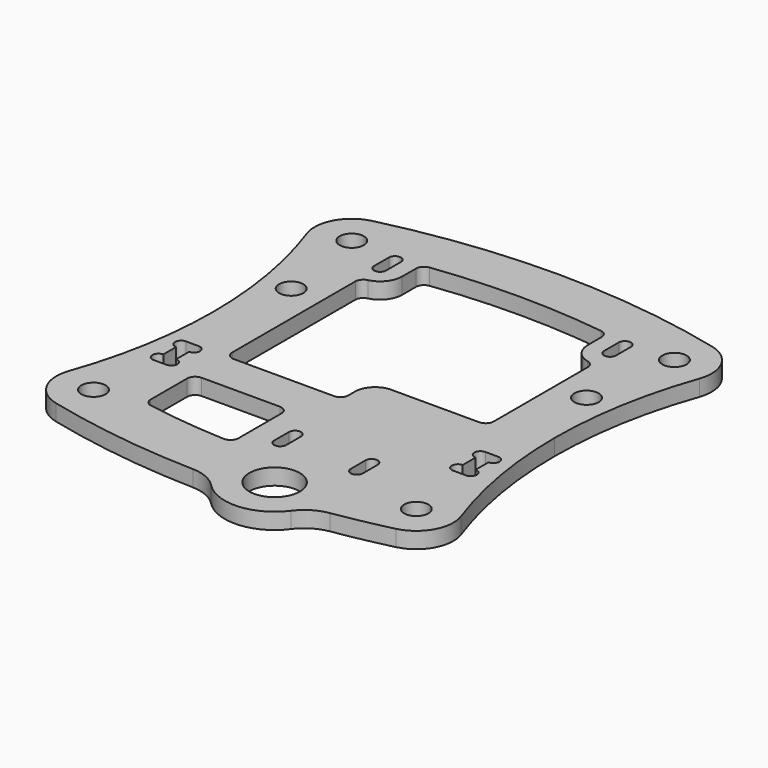
from build123d import *

# Parameters (mm, degrees)
F1_DEPTH  = 2
F3_DEPTH  = 2.001
F5_D      = 3
F8_DEPTH  = 2
F10_DEPTH = 2
F11_R     = 5
F13_DEPTH = 2.0010001
F14_R     = 3.125
F15_DEPTH = 2.0010001
F17_DEPTH = 2.0010001
F18_R     = 1
F19_R     = 2.5


# Not quite as in the source:
# - a feature names something its author has since deleted; it is built from what else it names


with BuildPart() as f1:
    # F0 (on Top) → F1 (new body)
    with BuildSketch(Plane.XY):
        with BuildLine():
            ThreePointArc((-18.4588585891, 24.3341531066), (-23.2526911935, 23.2526911935), (-24.3341531066, 18.4588585891))
            ThreePointArc((-24.3341531066, 18.4588585891), (-21.9518735553, 9.3657393117), (-21.15, 0))
            ThreePointArc((-21.15, 0), (-21.9518735553, -9.3657393117), (-24.3341531066, -18.4588585891))
            ThreePointArc((-24.3341531066, -18.4588585891), (-23.2526911935, -23.2526911935), (-18.4588585891, -24.3341531066))
            ThreePointArc((-18.4588585891, -24.3341531066), (-9.3657393117, -21.9518735553), (0, -21.15))
            ThreePointArc((0, -21.15), (9.3657393117, -21.9518735553), (18.4588585891, -24.3341531066))
            ThreePointArc((18.4588585891, -24.3341531066), (23.2526911935, -23.2526911935), (24.3341531066, -18.4588585891))
            ThreePointArc((24.3341531066, -18.4588585891), (21.9518735553, -9.3657393117), (21.15, 0))
            ThreePointArc((21.15, 0), (21.9518735553, 9.3657393117), (24.3341531066, 18.4588585891))
            ThreePointArc((24.3341531066, 18.4588585891), (23.2526911935, 23.2526911935), (18.4588585891, 24.3341531066))
            ThreePointArc((18.4588585891, 24.3341531066), (9.3657393117, 21.9518735553), (0, 21.15))
            ThreePointArc((0, 21.15), (-9.3657393117, 21.9518735553), (-18.4588585891, 24.3341531066))
        make_face()
    extrude(amount=F1_DEPTH)

    # F2 (on face) → F3 (cut, through all)
    with BuildSketch(Plane.XY.offset(2)):
        with BuildLine():
            Line((-18.55, -6.5), (-19.35, -6.5))
            ThreePointArc((-19.35, -6.5), (-20.1, -7.25), (-19.35, -8))
            Line((-19.35, -8), (-19.35, -9))
            Line((-19.35, -9), (-19.35, -10))
            ThreePointArc((-19.35, -10), (-20.1, -10.75), (-19.35, -11.5))
            Line((-19.35, -11.5), (-18.55, -11.5))
            Line((-18.55, -11.5), (-17.75, -11.5))
            ThreePointArc((-17.75, -11.5), (-17, -10.75), (-17.75, -10))
            Line((-17.75, -10), (-17.75, -9))
            Line((-17.75, -9), (-17.75, -8))
            ThreePointArc((-17.75, -8), (-17, -7.25), (-17.75, -6.5))
            Line((-17.75, -6.5), (-18.55, -6.5))
        make_face()
        with BuildLine():
            Line((18.55, -11.5), (19.35, -11.5))
            ThreePointArc((19.35, -11.5), (20.1, -10.75), (19.35, -10))
            Line((19.35, -10), (19.35, -9))
            Line((19.35, -9), (19.35, -8))
            ThreePointArc((19.35, -8), (20.1, -7.25), (19.35, -6.5))
            Line((19.35, -6.5), (18.55, -6.5))
            Line((18.55, -6.5), (17.75, -6.5))
            ThreePointArc((17.75, -6.5), (17, -7.25), (17.75, -8))
            Line((17.75, -8), (17.75, -9))
            Line((17.75, -9), (17.75, -10))
            ThreePointArc((17.75, -10), (17, -10.75), (17.75, -11.5))
            Line((17.75, -11.5), (18.55, -11.5))
        make_face()
    extrude(amount=-F3_DEPTH, mode=Mode.SUBTRACT)

    # F5 (through all)
    with Locations(Plane.XY.offset(2)):
        with Locations((-18.3, 8.5), (-20, 20), (20, 20), (18.3, 8.5), (20, -20), (-20, -20)):
            Hole(F5_D / 2)

    # F7 (on Top) → F8 (join, through all)
    with BuildSketch(Plane.XY):
        with BuildLine():
            ThreePointArc((21.0883280757, 24.4694006309), (10.6198106645, 26.3650888705), (0, 27))
            ThreePointArc((0, 27), (-10.6198106645, 26.3650888705), (-21.0883280757, 24.4694006309))
            ThreePointArc((-21.0883280757, 24.4694006309), (-19.7637100249, 24.5939271922), (-18.4588585891, 24.3341531066))
            ThreePointArc((-18.4588585891, 24.3341531066), (-9.3657393117, 21.9518735553), (0, 21.15))
            ThreePointArc((0, 21.15), (9.3657393117, 21.9518735553), (18.4588585891, 24.3341531066))
            ThreePointArc((18.4588585891, 24.3341531066), (19.7637100249, 24.5939271922), (21.0883280757, 24.4694006309))
        make_face()
    extrude(amount=F8_DEPTH)

    # F9 (on Top) → F10 (join, through all)
    with BuildSketch(Plane.XY):
        with BuildLine():
            ThreePointArc((11.6289429392, -26.2381484763), (16.3825233985, -25.4815286377), (21.0883280757, -24.4694006309))
            ThreePointArc((21.0883280757, -24.4694006309), (19.7637100249, -24.5939271922), (18.4588585891, -24.3341531066))
            ThreePointArc((18.4588585891, -24.3341531066), (9.3657393117, -21.9518735553), (0, -21.15))
            ThreePointArc((0, -21.15), (-9.3657393117, -21.9518735553), (-18.4588585891, -24.3341531066))
            ThreePointArc((-18.4588585891, -24.3341531066), (-19.7637100249, -24.5939271922), (-21.0883280757, -24.4694006309))
            ThreePointArc((-21.0883280757, -24.4694006309), (-10.4728212797, -26.3826037941), (0.2960579419, -26.9995083178))
            ThreePointArc((0.2960579419, -26.9995083178), (6.2139125454, -30.3611120266), (11.6289429392, -26.2381484763))
        make_face()
    extrude(amount=F10_DEPTH)

    # F11
    f11_edges = [f1.edges().sort_by_distance(p)[0] for p in [
        (0.296058, -26.999508, 1),
        (11.628943, -26.238148, 1),
    ]]
    fillet(f11_edges, radius=F11_R)

    # F12 (on face) → F13 (cut, through all)
    with BuildSketch(Plane.XY.offset(2)):
        with BuildLine():
            ThreePointArc((11.3, -15.1), (10.55, -14.35), (9.8, -15.1))
            Line((9.8, -15.1), (9.8, -17.4))
            ThreePointArc((9.8, -17.4), (10.55, -18.15), (11.3, -17.4))
            Line((11.3, -17.4), (11.3, -15.1))
        make_face()
        with BuildLine():
            ThreePointArc((1.8, -15.1), (1.05, -14.35), (0.3, -15.1))
            Line((0.3, -15.1), (0.3, -17.4))
            ThreePointArc((0.3, -17.4), (1.05, -18.15), (1.8, -17.4))
            Line((1.8, -17.4), (1.8, -15.1))
        make_face()
        with BuildLine():
            ThreePointArc((15, 19.5), (14.25, 20.25), (13.5, 19.5))
            Line((13.5, 19.5), (13.5, 17.2))
            ThreePointArc((13.5, 17.2), (14.25, 16.45), (15, 17.2))
            Line((15, 17.2), (15, 19.5))
        make_face()
        with BuildLine():
            ThreePointArc((-13.5, 19.5), (-14.25, 20.25), (-15, 19.5))
            Line((-15, 19.5), (-15, 17.2))
            ThreePointArc((-15, 17.2), (-14.25, 16.45), (-13.5, 17.2))
            Line((-13.5, 17.2), (-13.5, 19.5))
        make_face()
    extrude(amount=-F13_DEPTH, mode=Mode.SUBTRACT)

    # F14 (on face) → F15 (cut, through all)
    with BuildSketch(Plane.XY.offset(2)):
        with Locations((5.8, -24.2)):
            Circle(F14_R)
    extrude(amount=-F15_DEPTH, mode=Mode.SUBTRACT)

    # F16 (on face) → F17 (cut, through all)
    with BuildSketch(Plane.XY.offset(2)):
        with BuildLine():
            ThreePointArc((-11.5, 17.2), (-12.3592329599, 15.2031274452), (-14.4, 14.4540939565))
            Line((-14.4, 14.4540939565), (-14.4, -6.5))
            Line((-14.4, -6.5), (0, -6.5))
            Line((0, -6.5), (0, -2))
            Line((0, -2), (14.4, -2))
            Line((14.4, -2), (14.4, 14.4540939565))
            ThreePointArc((14.4, 14.4540939565), (12.3592329599, 15.2031274452), (11.5, 17.2))
            Line((11.5, 17.2), (11.5, 20.2007489844))
            ThreePointArc((11.5, 20.2007489844), (0, 21), (-11.5, 20.2007489844))
            Line((-11.5, 20.2007489844), (-11.5, 17.2))
        make_face()
        with BuildLine():
            ThreePointArc((-14.4, -18.9817306875), (-8.5718756396, -19.8028403577), (-2.7, -20.2057437268))
            Line((-2.7, -20.2057437268), (-2.7, -11.5))
            Line((-2.7, -11.5), (-14.4, -11.5))
            Line((-14.4, -11.5), (-14.4, -18.9817306875))
        make_face()
    extrude(amount=-F17_DEPTH, mode=Mode.SUBTRACT)

    # F18
    f18_edges = [f1.edges().sort_by_distance(p)[0] for p in [
        (-2.7, -11.5, 1),
        (-14.4, -11.5, 1),
        (-14.4, -18.981731, 1),
        (-2.7, -20.205744, 1),
        (11.5, 20.200749, 1),
        (-11.5, 20.200749, 1),
        (-14.4, -6.5, 1),
        (14.4, -2, 1),
        (0, -6.5, 1),
        (-14.4, 14.454094, 1),
        (14.4, 14.454094, 1),
    ]]
    fillet(f18_edges, radius=F18_R)

    # F19
    f19_edges = [f1.edges().sort_by_distance(p)[0] for p in [
        (0, -2, 1),
    ]]
    fillet(f19_edges, radius=F19_R)


solid = f1.part
